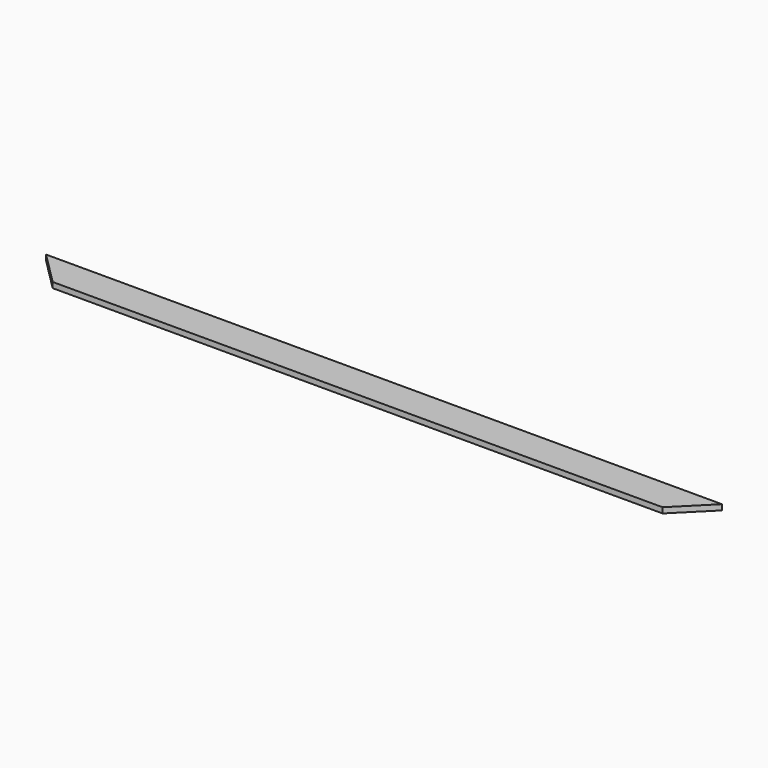
from build123d import *

# Parameters (mm, degrees)
F0_W     = 3124.2
F0_H     = 152.4
F1_DEPTH = 25.4
F2_SIZE  = 152.39999


# Not quite as in the source:
# - a fillet or chamfer is up to 0.001 mm smaller than in the source, because OpenCascade refuses the exact size


with BuildPart() as f1:
    # F0 (on Top) → F1 (new body)
    with BuildSketch(Plane.XY):
        with Locations((1562.1, -76.2)):
            Rectangle(F0_W, F0_H)
    extrude(amount=F1_DEPTH)

    # F2 (size 152.4 in the source; OpenCascade refuses exactly that, so slightly less here)
    f2_edges = [f1.edges().sort_by_distance(p)[0] for p in [
        (0, -152.4, 12.7),
        (3124.2, -152.4, 12.7),
    ]]
    chamfer(f2_edges, length=F2_SIZE)


solid = f1.part
